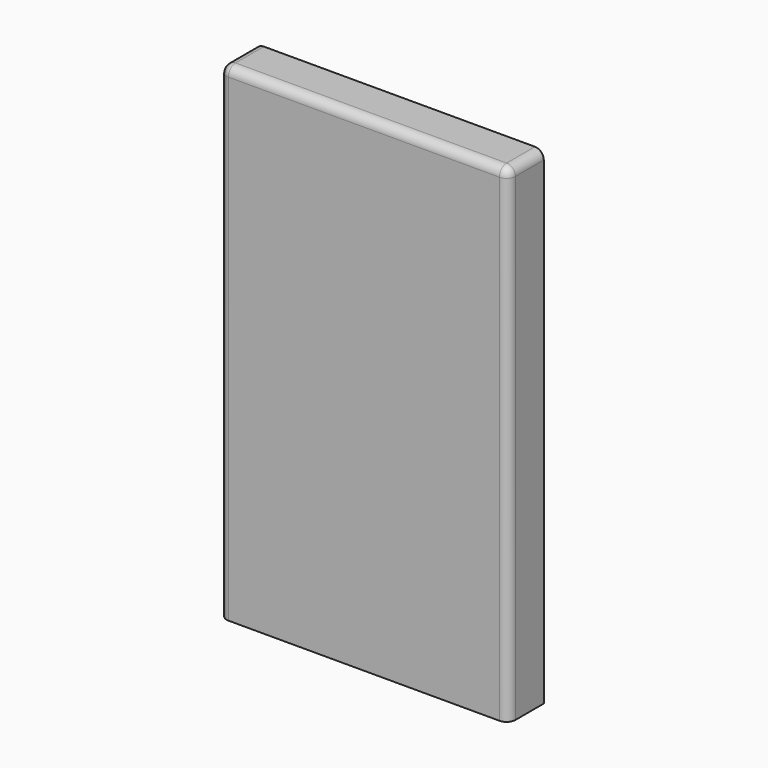
from build123d import *

# Parameters (mm, degrees)
F0_W     = 66.2185922265
F0_H     = 111.7807626724
F1_DEPTH = 10.16
F2_R     = 2.032
F3_T     = -4.064


# Not quite as in the source:
# - two fillets or chamfers of one size are made in one step


with BuildPart() as f1:
    # F0 (on Front) → F1 (new body)
    with BuildSketch(Plane.XZ):
        with Locations((-33.1092961133, 55.8903813362)):
            Rectangle(F0_W, F0_H)
    extrude(amount=F1_DEPTH)

    # F2
    f2_edges = [f1.edges().sort_by_distance(p)[0] for p in [
        (0, -10.16, 55.890381),
        (-66.218592, -10.16, 55.890381),
        (0, -5.08, 111.780763),
        (-66.218592, -5.08, 111.780763),
        (-33.109296, -10.16, 111.780763),
    ]]
    fillet(f2_edges, radius=F2_R)

    # F3
    f3_openings = [f1.faces().sort_by_distance(p)[0] for p in [
        (-33.109296, 0, 55.877105),
    ]]
    offset(amount=F3_T, openings=f3_openings)


solid = f1.part
